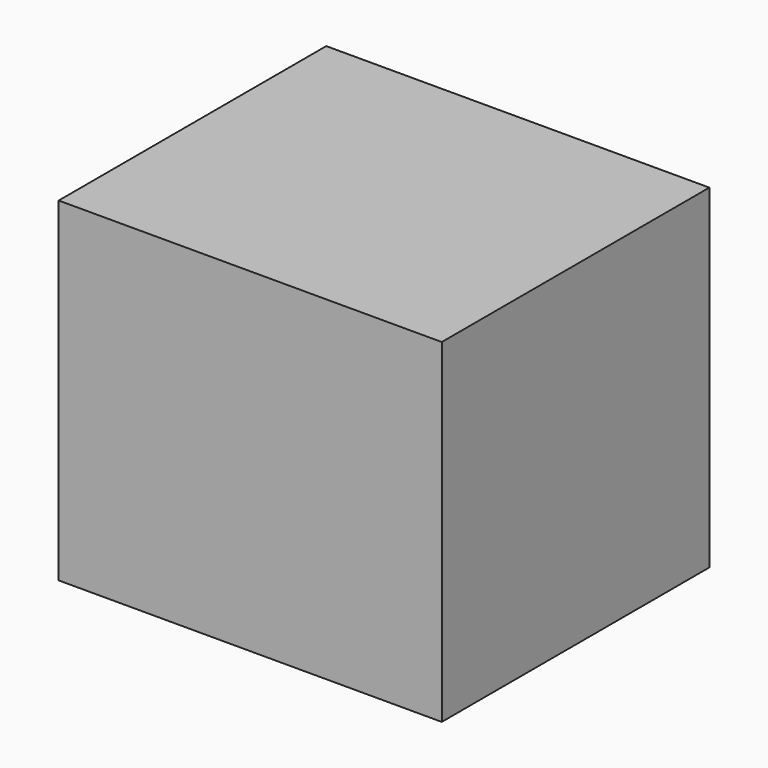
from build123d import *

# Parameters (mm, degrees)
F0_W     = 55
F0_H     = 55
F1_DEPTH = 63


# Not quite as in the source:
# - a feature names something its author has since deleted; it is built from what else it names


with BuildPart() as f1:
    # F0 (on Right) → F1 (new body)
    with BuildSketch(Plane.YZ):
        with Locations((98.5150450468, 41.700180769)):
            Rectangle(F0_W, F0_H)
    extrude(amount=F1_DEPTH)


solid = f1.part
